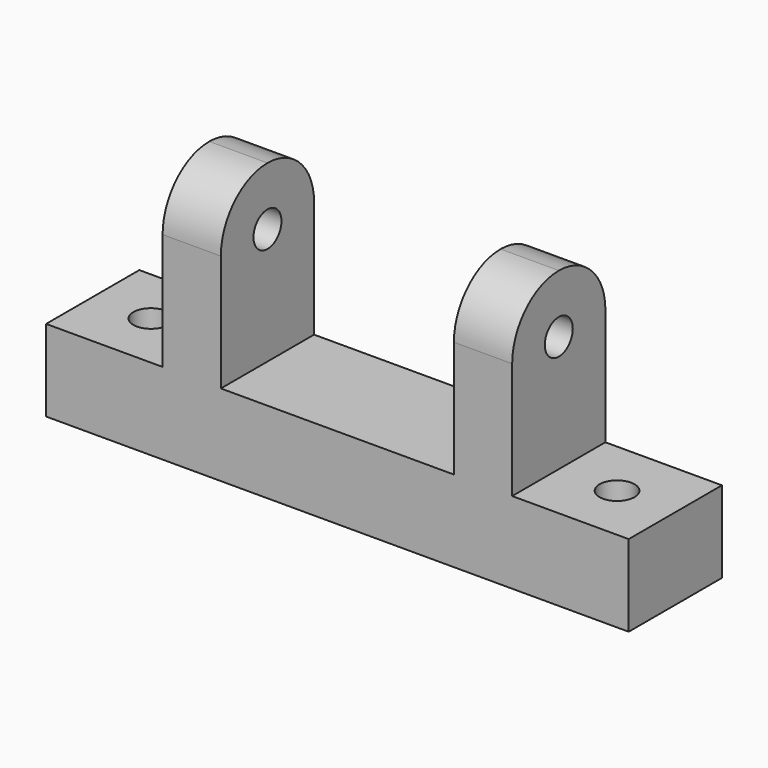
from build123d import *

# Parameters (mm, degrees)
F0_W      = 50
F0_H      = 10
F1_DEPTH  = 7
F2_W      = 30
F2_H      = 10
F4_DEPTH  = 15
F5_R      = 4.99999
F3_R      = 1.5
F6_DEPTH  = 25
F7_R      = 1.5
F8_DEPTH  = 50
F10_W     = 20
F10_H     = 10
F11_DEPTH = 25


# Not quite as in the source:
# - a fillet or chamfer is up to 0.001 mm smaller than in the source, because OpenCascade refuses the exact size


with BuildPart() as f1:
    # F0 (on Top) → F1 (new body)
    with BuildSketch(Plane.XY):
        with Locations((25, 5)):
            Rectangle(F0_W, F0_H)
    extrude(amount=F1_DEPTH)

    # F2 (on face) → F4 (join)
    with BuildSketch(Plane.XY.offset(7)):
        with Locations((25, 5)):
            Rectangle(F2_W, F2_H)
    extrude(amount=F4_DEPTH)

    # F5 (radius 5 in the source; OpenCascade refuses exactly that, so slightly less here)
    f5_edges = [f1.edges().sort_by_distance(p)[0] for p in [
        (25, 10, 22),
        (25, 0, 22),
    ]]
    fillet(f5_edges, radius=F5_R)

    # F3 (on face) → F6 (cut)
    with BuildSketch(Plane.XY.offset(7)):
        with Locations((45, 5)):
            Circle(F3_R)
        with Locations((5, 5)):
            Circle(F3_R)
    extrude(amount=-F6_DEPTH, mode=Mode.SUBTRACT)

    # F7 (on face) → F8 (cut)
    with BuildSketch(Plane.YZ.offset(40)):
        with Locations((5, 17)):
            Circle(F7_R)
    extrude(amount=-F8_DEPTH, mode=Mode.SUBTRACT)


with BuildPart() as f9_1:
    # F9: copy of F1
    add(f1.part.moved(Location((0, 0, 40))))

    # F10 (on face) → F11 (cut)
    with BuildSketch(Plane.XY.offset(47)):
        with Locations((25, 5)):
            Rectangle(F10_W, F10_H)
    extrude(amount=F11_DEPTH, mode=Mode.SUBTRACT)


solid = f9_1.part
